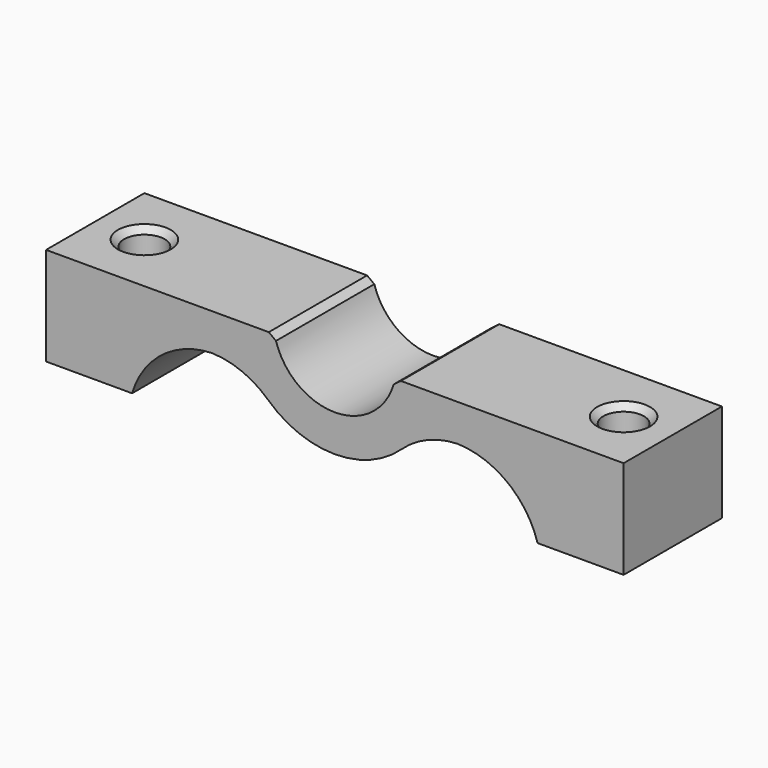
from build123d import *

# Parameters (mm, degrees)
F1_DEPTH    = 5
F3_T1_DEPTH = 5
F3_T3_DEPTH = 5
F4_T1_DEPTH = 6.2324692544
F4_T3_DEPTH = 6.2324692544
F2_R        = 1.65
F5_DEPTH    = 8.001
F6_SIZE     = 0.5


# Not quite as in the source:
# - a fillet or chamfer that OpenCascade refuses, or shapes differently, is made with other operations: its cross-section is extruded or revolved along the edge and cut away or added
# - a pattern or mirror of a feature is missing from the dataset's text; its kind, count and spacing are read off the source's solid


with BuildPart() as f1:
    # F0 (on Front) → F1 (new body, symmetric)
    with BuildSketch(Plane.XZ):
        with BuildLine():
            Line((23.5, -9), (23.5, -1))
            Line((23.5, -1), (4.8989794856, -1))
            ThreePointArc((4.8989794856, -1), (3.1622776602, -3.8729833462), (0, -5))
            ThreePointArc((0, -5), (-3.1622776602, -3.8729833462), (-4.8989794856, -1))
            Line((-4.8989794856, -1), (-23.5, -1))
            Line((-23.5, -1), (-23.5, -9))
            Line((-23.5, -9), (-16.5, -9))
            Line((-16.5, -9), (-16.5, -4))
            Line((-16.5, -4), (-6.9282032303, -4))
            ThreePointArc((-6.9282032303, -4), (-4, -6.9282032303), (0, -8))
            ThreePointArc((0, -8), (4, -6.9282032303), (6.9282032303, -4))
            Line((6.9282032303, -4), (16.5, -4))
            Line((16.5, -4), (16.5, -9))
            Line((16.5, -9), (23.5, -9))
        make_face()
    extrude(amount=F1_DEPTH, both=True)

    # F3: fillet of radius 7 on 8 edges, made by hand

    # F3_s2 → F3_t1 (join)
    with BuildSketch(Plane.XZ.offset(-5)):
        with BuildLine():
            ThreePointArc((9.7917960675, -4), (13.9750962002, -5.3875139198), (16.5, -9))
            Line((16.5, -9), (16.5, -4))
            Line((16.5, -4), (9.7917960675, -4))
        make_face()
        with BuildLine():
            ThreePointArc((5.4389541478, -5.8666666667), (7.6420004255, -4.4833546462), (10.1980390272, -4))
            Line((10.1980390272, -4), (6.9282032303, -4))
            ThreePointArc((6.9282032303, -4), (6.2536194731, -4.989212712), (5.4389541478, -5.8666666667))
        make_face()
        with BuildLine():
            ThreePointArc((-9.7917960675, -4), (-13.9750962002, -5.3875139198), (-16.5, -9))
            Line((-16.5, -9), (-16.5, -4))
            Line((-16.5, -4), (-9.7917960675, -4))
        make_face()
        with BuildLine():
            ThreePointArc((-5.4389541478, -5.8666666667), (-7.6420004255, -4.4833546462), (-10.1980390272, -4))
            Line((-10.1980390272, -4), (-6.9282032303, -4))
            ThreePointArc((-6.9282032303, -4), (-6.2536194731, -4.989212712), (-5.4389541478, -5.8666666667))
        make_face()
    extrude(amount=F3_T1_DEPTH)

    # F3_s4 → F3_t3 (join)
    with BuildSketch(Plane.XZ):
        with BuildLine():
            ThreePointArc((9.7917960675, -4), (13.9750962002, -5.3875139198), (16.5, -9))
            Line((16.5, -9), (16.5, -4))
            Line((16.5, -4), (9.7917960675, -4))
        make_face()
        with BuildLine():
            ThreePointArc((5.4389541478, -5.8666666667), (7.6420004255, -4.4833546462), (10.1980390272, -4))
            Line((10.1980390272, -4), (6.9282032303, -4))
            ThreePointArc((6.9282032303, -4), (6.2536194731, -4.989212712), (5.4389541478, -5.8666666667))
        make_face()
        with BuildLine():
            ThreePointArc((-9.7917960675, -4), (-13.9750962002, -5.3875139198), (-16.5, -9))
            Line((-16.5, -9), (-16.5, -4))
            Line((-16.5, -4), (-9.7917960675, -4))
        make_face()
        with BuildLine():
            ThreePointArc((-5.4389541478, -5.8666666667), (-7.6420004255, -4.4833546462), (-10.1980390272, -4))
            Line((-10.1980390272, -4), (-6.9282032303, -4))
            ThreePointArc((-6.9282032303, -4), (-6.2536194731, -4.989212712), (-5.4389541478, -5.8666666667))
        make_face()
    extrude(amount=F3_T3_DEPTH)

    # F4: chamfer of 0.5 on 4 edges, made by hand

    # F4_s2 → F4_t1 (cut)
    with BuildSketch(Plane.XZ.offset(-6.2324692544)):
        with BuildLine():
            Line((-4.7731743681, -1.4483837223), (-5.3918225964, -0.9880608955))
            Line((-5.3918225964, -0.9880608955), (-5.3918225964, -0.9780608955))
            ThreePointArc((-5.3918225964, -0.9780608955), (-5.145401041, -0.99), (-4.8989794856, -0.99))
            Line((-4.8989794856, -0.99), (-4.8891815266, -0.998))
            ThreePointArc((-4.8891815266, -0.998), (-4.8374189809, -1.2245315852), (-4.7635959284, -1.445510833))
            Line((-4.7635959284, -1.445510833), (-4.7731743681, -1.4483837223))
        make_face()
        with BuildLine():
            Line((5.3918225964, -0.9880608955), (4.7731743681, -1.4483837223))
            Line((4.7731743681, -1.4483837223), (4.7635959284, -1.445510833))
            ThreePointArc((4.7635959284, -1.445510833), (4.8374189809, -1.2245315852), (4.8891815266, -0.998))
            Line((4.8891815266, -0.998), (4.8989794856, -0.99))
            ThreePointArc((4.8989794856, -0.99), (5.145401041, -0.99), (5.3918225964, -0.9780608955))
            Line((5.3918225964, -0.9780608955), (5.3918225964, -0.9880608955))
        make_face()
    extrude(amount=F4_T1_DEPTH, mode=Mode.SUBTRACT)

    # F4_s4 → F4_t3 (cut)
    with BuildSketch(Plane.XZ):
        with BuildLine():
            Line((-4.7731743681, -1.4483837223), (-5.3918225964, -0.9880608955))
            Line((-5.3918225964, -0.9880608955), (-5.3918225964, -0.9780608955))
            ThreePointArc((-5.3918225964, -0.9780608955), (-5.145401041, -0.99), (-4.8989794856, -0.99))
            Line((-4.8989794856, -0.99), (-4.8891815266, -0.998))
            ThreePointArc((-4.8891815266, -0.998), (-4.8374189809, -1.2245315852), (-4.7635959284, -1.445510833))
            Line((-4.7635959284, -1.445510833), (-4.7731743681, -1.4483837223))
        make_face()
        with BuildLine():
            Line((5.3918225964, -0.9880608955), (4.7731743681, -1.4483837223))
            Line((4.7731743681, -1.4483837223), (4.7635959284, -1.445510833))
            ThreePointArc((4.7635959284, -1.445510833), (4.8374189809, -1.2245315852), (4.8891815266, -0.998))
            Line((4.8891815266, -0.998), (4.8989794856, -0.99))
            ThreePointArc((4.8989794856, -0.99), (5.145401041, -0.99), (5.3918225964, -0.9780608955))
            Line((5.3918225964, -0.9780608955), (5.3918225964, -0.9880608955))
        make_face()
    extrude(amount=F4_T3_DEPTH, mode=Mode.SUBTRACT)

    # F2 (on face) → F5 (cut, through all)
    with BuildSketch(Plane(origin=(0, 0, -9), x_dir=(1, 0, 0), z_dir=(0, 0, -1))):
        with Locations((19.5, 0)):
            Circle(F2_R)
    f5 = extrude(amount=-F5_DEPTH, mode=Mode.SUBTRACT)

    # F5_copies: F5 across plane
    add(f5.mirror(Plane(origin=(0, 0, 0), x_dir=(0, 0, -1), z_dir=(-1, 0, 0))), mode=Mode.SUBTRACT)

    # F6
    f6_edges = [f1.edges().sort_by_distance(p)[0] for p in [
        (19.5, 1.65, -9),
        (19.5, -1.65, -9),
        (19.5, 1.65, -1),
        (-19.5, 1.65, -9),
        (-19.5, 1.65, -1),
        (-19.5, -1.65, -9),
        (-19.5, -1.65, -1),
        (19.5, -1.65, -1),
    ]]
    chamfer(f6_edges, length=F6_SIZE)


solid = f1.part
